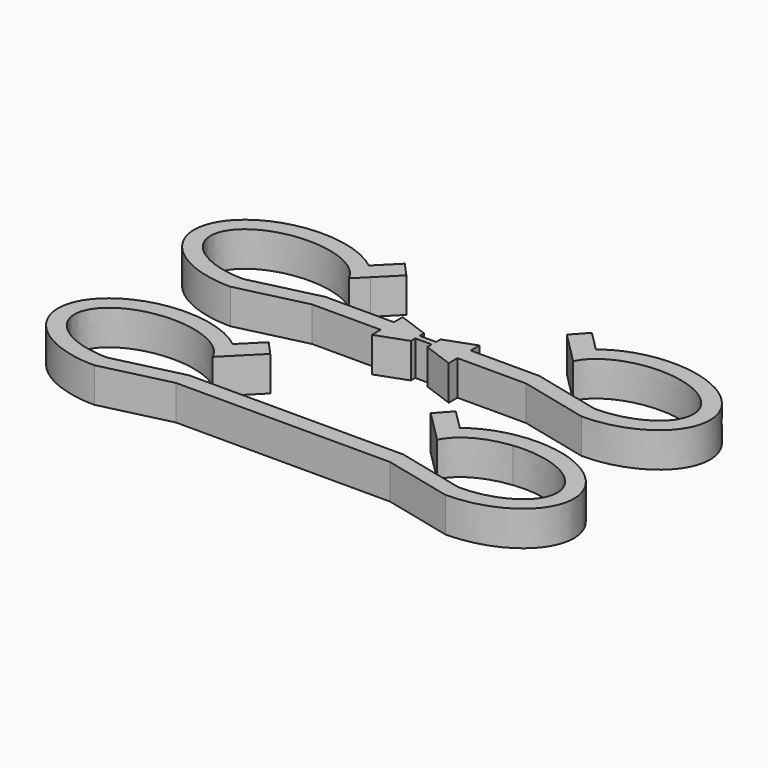
from build123d import *

# Parameters (mm, degrees)
F1_DEPTH = 6.35
F2_DEPTH = 6.35


# Not quite as in the source:
# - ends of sketch curves that miss each other by under 0.0002 mm in the source are joined


with BuildPart() as f1:
    # F0 (on Top) → F1 (new body)
    with BuildSketch(Plane.XY):
        with BuildLine():
            add(Edge.make_bspline(
                [(-20.4512735689, -13.4928953942), (-27.006583317, 1.0216576775), (-41.568666167, -11.0043361613), (-56.130749017, -23.03033), (-32, -23.03033)],
                knots=[3.416708, 3.416708, 3.416708, 5.635344817, 5.635344817, 7.853981634, 7.853981634, 7.853981634], degree=2, weights=[1, 0.445271914, 1, 0.445271914, 1]))
            Line((-20.4512735689, -13.4928953942), (-14.623441, -7.659787))
            Line((-14.623441, -7.659787), (-17.0484084715, -4.9831928082))
            Line((-17.0484084715, -4.9831928082), (-20.6942287896, -8.6297607204))
            add(Edge.make_bspline(
                [(-20.6942287896, -8.6297607204), (-20.698607878, -8.6262451494), (-20.7029914266, -8.6227323031)],
                knots=[3.8586865618, 3.8586865618, 3.8586865618, 3.859575, 3.859575, 3.859575], degree=2, weights=[1, 0.9999999013, 1]))
            add(Edge.make_bspline(
                [(-20.7029914266, -8.6227323031), (-36.0243090451, 3.6553185791), (-45.6568538904, -11.1875086941), (-55.2893987358, -26.0303359672), (-31.9999945096, -26.03033)],
                knots=[3.859575, 3.859575, 3.859575, 5.8567785, 5.8567785, 7.853982, 7.853982, 7.853982], degree=2, weights=[1, 0.5414783641, 1, 0.5414783641, 1]))
            Line((-31.9999945096, -26.03033), (-19.5, -23.03033))
            Line((-19.5, -23.03033), (0, -23.03033))
            Line((0, -23.03033), (19.5, -23.03033))
            Line((19.5, -23.03033), (32, -26.03033))
            add(Edge.make_bspline(
                [(32, -26.03033), (46.9999832548, -26.0303338433), (46.999986, -15.5303319216), (46.9999887452, -5.03033), (32, -5.03033)],
                knots=[4.7123886144, 4.7123886144, 4.7123886144, 6.2831851242, 6.2831851242, 7.853981634, 7.853981634, 7.853981634], degree=2, weights=[1, 0.7071067165, 1, 0.7071067165, 1]))
            add(Edge.make_bspline(
                [(32, -5.03033), (25.1858150627, -5.03033), (20.7029914266, -8.6227323031)],
                knots=[1.5707963268, 1.5707963268, 1.5707963268, 2.4236103072, 2.4236103072, 2.4236103072], degree=2, weights=[1, 0.9104577001, 1]))
            add(Edge.make_bspline(
                [(20.7029914266, -8.6227323031), (20.698607878, -8.6262451494), (20.6942287896, -8.6297607204)],
                knots=[2.4236103072, 2.4236103072, 2.4236103072, 2.4244987453, 2.4244987453, 2.4244987453], degree=2, weights=[1, 0.9999999013, 1]))
            Line((20.6942287896, -8.6297607204), (17.0484127896, -4.9831967204))
            Line((17.0484127896, -4.9831967204), (14.623441, -7.659787))
            Line((14.623441, -7.659787), (20.4512735689, -13.4928953942))
            add(Edge.make_bspline(
                [(30.0004237684, -8.1351855073), (22.5138875018, -8.9259228869), (20.4512735689, -13.4928953942)],
                knots=[1.7382085912, 1.7382085912, 1.7382085912, 2.8664773072, 2.8664773072, 2.8664773072], degree=2, weights=[1, 0.8450517623, 1]))
            add(Edge.make_bspline(
                [(32, -8.03033), (30.9931737994, -8.03033), (30.0004237684, -8.1351855073)],
                knots=[1.5707963268, 1.5707963268, 1.5707963268, 1.7382085912, 1.7382085912, 1.7382085912], degree=2, weights=[1, 0.9964986868, 1]))
            add(Edge.make_bspline(
                [(32, -23.03033), (44, -23.03033), (44, -15.53033), (44, -8.03033), (32, -8.03033)],
                knots=[4.7123889804, 4.7123889804, 4.7123889804, 6.2831853072, 6.2831853072, 7.853981634, 7.853981634, 7.853981634], degree=2, weights=[1, 0.7071067812, 1, 0.7071067812, 1]))
            Line((32, -23.03033), (19.5000043923, -20.03033))
            Line((19.5000043923, -20.03033), (0, -20.03033))
            Line((0, -20.03033), (-19.5, -20.03033))
            Line((-19.5, -20.03033), (-32, -23.03033))
        make_face()
    extrude(amount=F1_DEPTH)


with BuildPart() as f2:
    # F0 (on Top) → F2 (new body)
    with BuildSketch(Plane.XY):
        with BuildLine():
            add(Edge.make_bspline(
                [(-18.2670631482, 19.6932923503), (-18.2676990936, 19.69430555), (-18.2683353441, 19.6953186559)],
                knots=[3.5555654943, 3.5555654943, 3.5555654943, 3.5557762907, 3.5557762907, 3.5557762907], degree=2, weights=[1, 0.9999999944, 1]))
            Line((-18.2683353441, 19.6953186559), (-14.623441, 23.340213))
            Line((-14.623441, 23.340213), (-17.0484127896, 26.0168032796))
            Line((-17.0484127896, 26.0168032796), (-20.6942287896, 22.3702392796))
            add(Edge.make_bspline(
                [(-20.6942287896, 22.3702392796), (-20.698607878, 22.3737548506), (-20.7029914266, 22.3772676969)],
                knots=[3.8586865618, 3.8586865618, 3.8586865618, 3.859575, 3.859575, 3.859575], degree=2, weights=[1, 0.9999999013, 1]))
            add(Edge.make_bspline(
                [(-20.7029914266, 22.3772676969), (-36.0243090451, 34.6553185791), (-45.6568538904, 19.8124913059), (-55.2893987358, 4.9696640328), (-31.9999945096, 4.96967)],
                knots=[3.859575, 3.859575, 3.859575, 5.8567785, 5.8567785, 7.853982, 7.853982, 7.853982], degree=2, weights=[1, 0.5414783641, 1, 0.5414783641, 1]))
            Line((-31.9999945096, 4.96967), (-19.5, 7.96967))
            Line((-19.5, 7.96967), (-7, 7.96967))
            Line((-7, 7.96967), (-7, 5.96967))
            Line((-7, 5.96967), (-1.5, 7.96967))
            Line((-1.5, 7.96967), (-1.5, 8.96967))
            Line((-1.5, 8.96967), (0, 8.96967))
            Line((0, 8.96967), (1.5, 8.96967))
            Line((1.5, 8.96967), (1.5, 7.96967))
            Line((1.5, 7.96967), (7, 5.96967))
            Line((7, 5.96967), (7, 7.96967))
            Line((7, 7.96967), (19.5, 7.96967))
            Line((19.5, 7.96967), (32, 4.96967))
            add(Edge.make_bspline(
                [(32, 4.96967), (55.2893995447, 4.96967), (45.656852755, 19.8124930555), (36.0243059653, 34.655316111), (20.7029914266, 22.3772676969)],
                knots=[4.7123889804, 4.7123889804, 4.7123889804, 6.7095922974, 6.7095922974, 8.7067956144, 8.7067956144, 8.7067956144], degree=2, weights=[1, 0.541478441, 1, 0.541478441, 1]))
            add(Edge.make_bspline(
                [(20.7029914266, 22.3772676969), (20.698607878, 22.3737548506), (20.6942287896, 22.3702392796)],
                knots=[2.4236103072, 2.4236103072, 2.4236103072, 2.4244987453, 2.4244987453, 2.4244987453], degree=2, weights=[1, 0.9999999013, 1]))
            Line((20.6942287896, 22.3702392796), (17.0484127896, 26.0168032796))
            Line((17.0484127896, 26.0168032796), (14.6234453181, 23.3402090878))
            Line((14.6234453181, 23.3402090878), (20.4512735689, 17.5071046058))
            add(Edge.make_bspline(
                [(32, 7.96967), (56.130749017, 7.96967), (41.568666167, 19.9956638387), (27.006583317, 32.0216576775), (20.4512735689, 17.5071046058)],
                knots=[4.7123889804, 4.7123889804, 4.7123889804, 6.9310257974, 6.9310257974, 9.1496626144, 9.1496626144, 9.1496626144], degree=2, weights=[1, 0.445271914, 1, 0.445271914, 1]))
            Line((32, 7.96967), (19.5, 10.96967))
            Line((19.5, 10.96967), (7, 10.96967))
            Line((7, 10.96967), (7, 12.96967))
            Line((7, 12.96967), (1.5, 10.96967))
            Line((1.5, 10.96967), (1.5, 9.96967))
            Line((1.5, 9.96967), (0, 9.96967))
            Line((0, 9.96967), (-1.5, 9.96967))
            Line((-1.5, 9.96967), (-1.5, 10.96967))
            Line((-1.5, 10.96967), (-7, 12.96967))
            Line((-7, 12.96967), (-7, 10.96967))
            Line((-7, 10.96967), (-19.5, 10.96967))
            Line((-19.5, 10.96967), (-32, 7.96967))
            add(Edge.make_bspline(
                [(-20.4512735689, 17.5071046058), (-27.006583317, 32.0216576775), (-41.568666167, 19.9956638387), (-56.130749017, 7.96967), (-32, 7.96967)],
                knots=[3.416708, 3.416708, 3.416708, 5.635344817, 5.635344817, 7.853981634, 7.853981634, 7.853981634], degree=2, weights=[1, 0.445271914, 1, 0.445271914, 1]))
            Line((-20.4512735689, 17.5071046058), (-18.2670631482, 19.6932923503))
        make_face()
    extrude(amount=F2_DEPTH)


solid = Compound([f1.part, f2.part])
